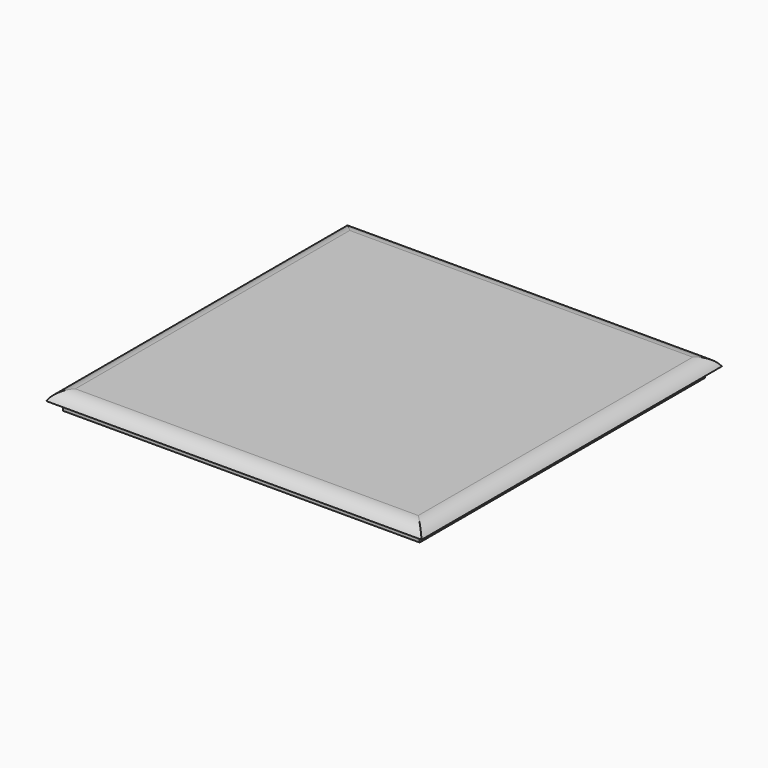
from build123d import *

# Parameters (mm, degrees)
F1_W        = 101.6
F1_H        = 101.6
F1_W_2      = 96.52
F1_H_2      = 96.52
F2_DEPTH    = 2.54
F3_T1_DEPTH = 123.5970452561
F3_T3_DEPTH = 123.5970452561
F4_DEPTH    = 2.54


# Not quite as in the source:
# - a fillet or chamfer that OpenCascade refuses, or shapes differently, is made with other operations: its cross-section is extruded or revolved along the edge and cut away or added


with BuildPart() as f2:
    # F1 (on offset) → F2 (new body)
    with BuildSketch(Plane.XY.offset(101.6)):
        with Locations((-130.4673959928, -63.7241914409)):
            Rectangle(F1_W, F1_H)
        with Locations((-130.4673959928, -63.7241914409)):
            Rectangle(F1_W_2, F1_H_2, mode=Mode.SUBTRACT)
        with Locations((-130.4673959928, -63.7241914409)):
            Rectangle(F1_W_2, F1_H_2)
    extrude(amount=F2_DEPTH)

    # F3: fillet of radius 5.08 on 4 edges, made by hand

    # F3_s2 → F3_t1 (cut)
    with BuildSketch(Plane.YZ.offset(-192.2659186209)):
        with BuildLine():
            ThreePointArc((-114.5241914409, 101.6), (-112.6647823896, 103.4594090512), (-110.1247823896, 104.14))
            Line((-110.1247823896, 104.14), (-114.5241914409, 104.14))
            Line((-114.5241914409, 104.14), (-114.5241914409, 101.6))
        make_face()
        with BuildLine():
            ThreePointArc((-12.9241914409, 101.6), (-14.7836004921, 103.4594090512), (-17.3236004921, 104.14))
            Line((-17.3236004921, 104.14), (-12.9241914409, 104.14))
            Line((-12.9241914409, 104.14), (-12.9241914409, 101.6))
        make_face()
    extrude(amount=F3_T1_DEPTH, mode=Mode.SUBTRACT)

    # F3_s4 → F3_t3 (cut)
    with BuildSketch(Plane.XZ.offset(1.9256688128)):
        with BuildLine():
            ThreePointArc((-79.6673959928, 101.6), (-81.526805044, 103.4594090512), (-84.066805044, 104.14))
            Line((-84.066805044, 104.14), (-79.6673959928, 104.14))
            Line((-79.6673959928, 104.14), (-79.6673959928, 101.6))
        make_face()
        with BuildLine():
            ThreePointArc((-181.2673959928, 101.6), (-179.4079869416, 103.4594090512), (-176.8679869416, 104.14))
            Line((-176.8679869416, 104.14), (-181.2673959928, 104.14))
            Line((-181.2673959928, 104.14), (-181.2673959928, 101.6))
        make_face()
    extrude(amount=F3_T3_DEPTH, mode=Mode.SUBTRACT)

    # F1 (on offset) → F4 (join)
    with BuildSketch(Plane.XY.offset(101.6)):
        with Locations((-130.4673959928, -63.7241914409)):
            Rectangle(F1_W_2, F1_H_2)
    extrude(amount=-F4_DEPTH)


solid = f2.part
